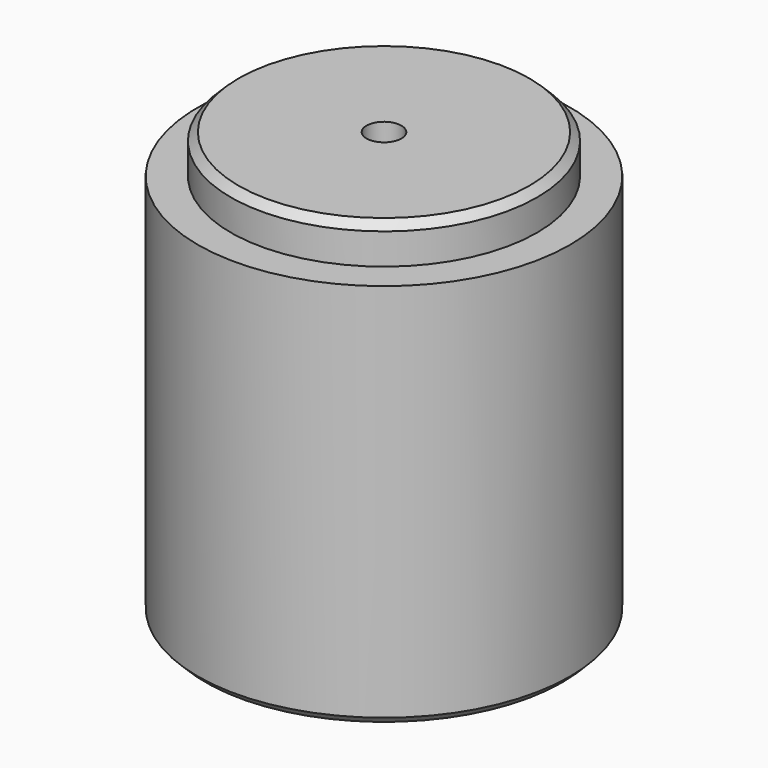
from build123d import *

# Parameters (mm, degrees)
F0_R     = 24
F1_DEPTH = 50
F2_R     = 19.75
F3_DEPTH = 5
F4_R     = 7.5
F5_DEPTH = 45
F6_R     = 2.25
F7_DEPTH = 10
F8_SIZE  = 1
F9_SIZE  = 5.24999


# Not quite as in the source:
# - a fillet or chamfer is up to 0.001 mm smaller than in the source, because OpenCascade refuses the exact size


with BuildPart() as f1:
    # F0 (on Top) → F1 (new body)
    with BuildSketch(Plane.XY):
        Circle(F0_R)
    extrude(amount=F1_DEPTH)

    # F2 (on face) → F3 (join)
    with BuildSketch(Plane.XY.offset(50)):
        Circle(F2_R)
    extrude(amount=F3_DEPTH)

    # F4 (on face) → F5 (cut)
    with BuildSketch(Plane(origin=(0, 0, 0), x_dir=(1, 0, 0), z_dir=(0, 0, -1))):
        Circle(F4_R)
    extrude(amount=-F5_DEPTH, mode=Mode.SUBTRACT)

    # F6 (on face) → F7 (cut)
    with BuildSketch(Plane(origin=(0, 0, 45), x_dir=(1, 0, 0), z_dir=(0, 0, -1))):
        Circle(F6_R)
    extrude(amount=-F7_DEPTH, mode=Mode.SUBTRACT)

    # F8
    f8_edges = [f1.edges().sort_by_distance(p)[0] for p in [
        (-24, 0, 0),
        (-7.5, 0, 0),
        (-19.75, 0, 55),
    ]]
    chamfer(f8_edges, length=F8_SIZE)

    # F9 (size 5.25 in the source; OpenCascade refuses exactly that, so slightly less here)
    f9_edges = [f1.edges().sort_by_distance(p)[0] for p in [
        (-7.5, 0, 45),
    ]]
    chamfer(f9_edges, length=F9_SIZE)


solid = f1.part
